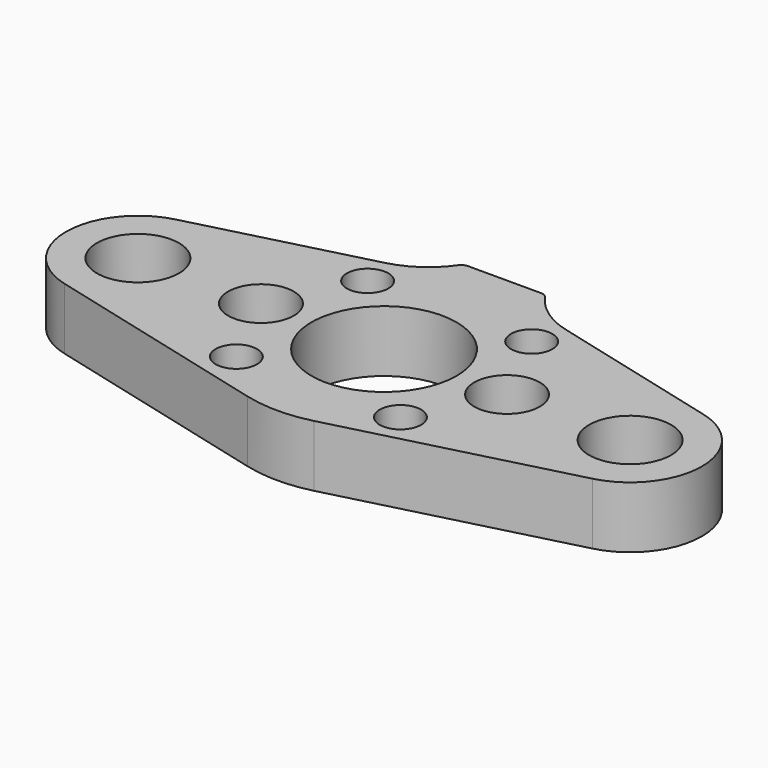
from build123d import *

# Parameters (mm, degrees)
F0_R        = 3.2004
F0_R_2      = 6.35
F0_R_3      = 5.08
F0_R_4      = 11.2395
F1_DEPTH    = 9.525
F2_W        = 12.7
F2_H        = 5.1071889116
F3_DEPTH    = 9.525
F4_T1_DEPTH = 9.525
F5_R        = 1.27


# Not quite as in the source:
# - a fillet or chamfer that OpenCascade refuses, or shapes differently, is made with other operations: its cross-section is extruded or revolved along the edge and cut away or added


with BuildPart() as f1:
    # F0 (on Top) → F1 (new body)
    with BuildSketch(Plane.XY):
        with BuildLine():
            Line((-5.159375, 19.9821734518), (-40.878125, 10.7596318587))
            ThreePointArc((-40.878125, 10.7596318587), (-49.2125, 0), (-40.878125, -10.7596318587))
            Line((-40.878125, -10.7596318587), (-5.159375, -19.9821734518))
            ThreePointArc((-5.159375, -19.9821734518), (0, -20.6375), (5.159375, -19.9821734518))
            Line((5.159375, -19.9821734518), (40.878125, -10.7596318587))
            ThreePointArc((40.878125, -10.7596318587), (49.2125, 0), (40.878125, 10.7596318587))
            Line((40.878125, 10.7596318587), (5.159375, 19.9821734518))
            ThreePointArc((5.159375, 19.9821734518), (0, 20.6375), (-5.159375, 19.9821734518))
        make_face()
        with Locations((-12.7, -12.7)):
            Circle(F0_R, mode=Mode.SUBTRACT)
        with Locations((12.7, -12.7)):
            Circle(F0_R, mode=Mode.SUBTRACT)
        with Locations((-38.1, 0)):
            Circle(F0_R_2, mode=Mode.SUBTRACT)
        with Locations((-19.05, 0)):
            Circle(F0_R_3, mode=Mode.SUBTRACT)
        with Locations((-12.7, 12.7)):
            Circle(F0_R, mode=Mode.SUBTRACT)
        Circle(F0_R_4, mode=Mode.SUBTRACT)
        with Locations((19.05, 0)):
            Circle(F0_R_3, mode=Mode.SUBTRACT)
        with Locations((38.1, 0)):
            Circle(F0_R_2, mode=Mode.SUBTRACT)
        with Locations((12.7, 12.7)):
            Circle(F0_R, mode=Mode.SUBTRACT)
    extrude(amount=F1_DEPTH)

    # F2 (on face) → F3 (join, through all)
    with BuildSketch(Plane.XY.offset(9.525)):
        with Locations((0, 20.7509055442)):
            Rectangle(F2_W, F2_H)
    extrude(amount=-F3_DEPTH)

    # F4: fillet of radius 12.7 on 2 edges, made by hand

    # F4_s2 → F4_t1 (join)
    with BuildSketch(Plane.XY):
        with BuildLine():
            ThreePointArc((-13.9630832797, 17.7090657484), (-9.6168370541, 19.7724670423), (-6.35, 23.3045))
            Line((-6.35, 23.3045), (-6.35, 19.6747553987))
            Line((-6.35, 19.6747553987), (-13.9630832797, 17.7090657484))
        make_face()
        with BuildLine():
            ThreePointArc((13.9630832797, 17.7090657484), (9.6168370541, 19.7724670423), (6.35, 23.3045))
            Line((6.35, 23.3045), (6.35, 19.6747553987))
            Line((6.35, 19.6747553987), (13.9630832797, 17.7090657484))
        make_face()
    extrude(amount=F4_T1_DEPTH)

    # F5
    f5_edges = [f1.edges().sort_by_distance(p)[0] for p in [
        (-6.35, 23.3045, 4.7625),
        (6.35, 23.3045, 4.7625),
    ]]
    fillet(f5_edges, radius=F5_R)


solid = f1.part
